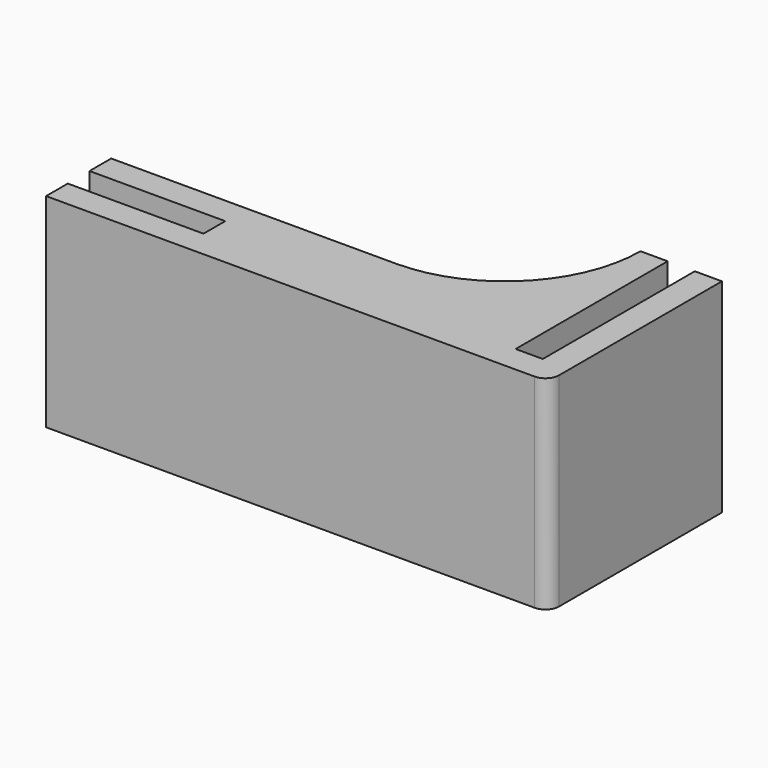
from build123d import *

# Parameters (mm, degrees)
F1_DEPTH = 7.5
F2_R     = 9.99999
F3_R     = 1


# Not quite as in the source:
# - a fillet or chamfer is up to 0.001 mm smaller than in the source, because OpenCascade refuses the exact size


with BuildPart() as f1:
    # F0 (on Top) → F1 (new body, symmetric)
    with BuildSketch(Plane.XY):
        Polygon((-9.7452771891, 18.3048394923), (-9.7452771891, 8.3048394923), (-40.7452771891, 8.3048394923), (-40.7452771891, 6.3048394923), (-30.7452771891, 6.3048394923), (-30.7452771891, 4.3048394923), (-40.7452771891, 4.3048394923), (-40.7452771891, 2.3048394923), (-3.7452771891, 2.3048394923), (-3.7452771891, 18.3048394923), (-5.7452771891, 18.3048394923), (-5.7452771891, 4.3048394923), (-7.7452771891, 4.3048394923), (-7.7452771891, 18.3048394923), align=None)
    extrude(amount=F1_DEPTH, both=True)

    # F2 (radius 10 in the source; OpenCascade refuses exactly that, so slightly less here)
    f2_edges = [f1.edges().sort_by_distance(p)[0] for p in [
        (-9.745277, 8.304839, 0),
    ]]
    fillet(f2_edges, radius=F2_R)

    # F3
    f3_edges = [f1.edges().sort_by_distance(p)[0] for p in [
        (-3.745277, 2.304839, 0),
    ]]
    fillet(f3_edges, radius=F3_R)


solid = f1.part
